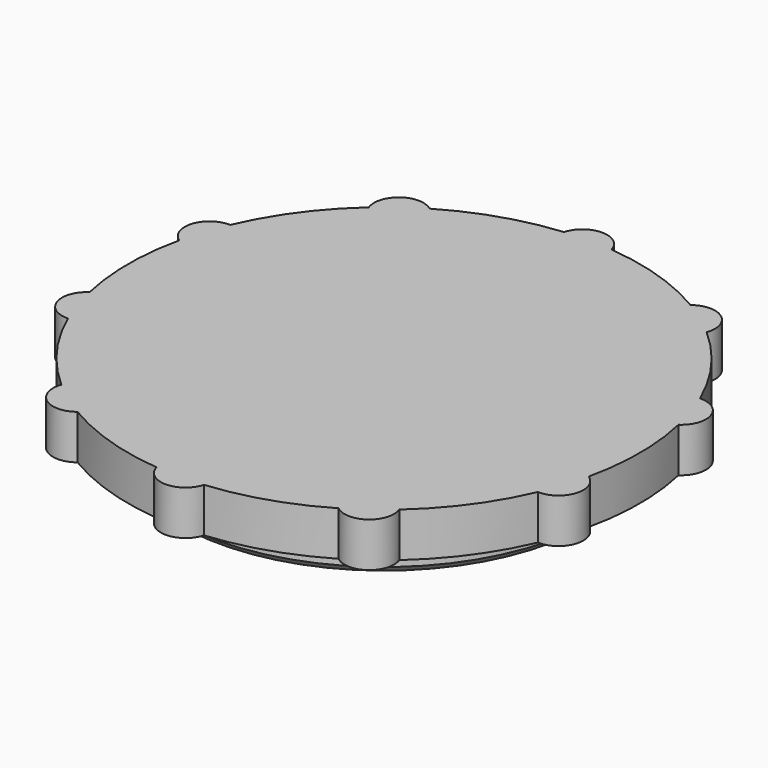
from build123d import *

# Parameters (mm, degrees)
F3_R            = 1.4097
F4_DEPTH        = 2.54
F4_COPIES_COUNT = 10
F5_SIZE         = 0.381


# Not quite as in the source:
# - a pattern or mirror of a feature is missing from the dataset's text; its kind, count and spacing are read off the source's solid


with BuildPart() as f2:
    # F1 (on Front) → F2 (revolve)
    with BuildSketch(Plane.XZ):
        Polygon((-14.605, 0), (-12.0904, 0), (-12.0904, -2.032), (-10.5791, -2.032), (-10.5791, 0), (-8.763, 0), (-7.874, 1.524), (0, 1.524), (0, 2.54), (-14.605, 2.54), align=None)
    revolve(axis=Axis((0, 0, -1.27), (0, 0, -1)))

    # F3 (on face) → F4 (join, through all)
    with BuildSketch(Plane.XY.offset(2.54)):
        with Locations((0, 14.1607994729)):
            Circle(F3_R)
    f4 = extrude(amount=-F4_DEPTH)

    # F4_copies: F4 ×10 about axis
    f4_copies_axis = Axis((0, 0, 0), (0, 0, 1))
    for i in range(1, F4_COPIES_COUNT):
        add(f4.rotate(f4_copies_axis, i * 360 / F4_COPIES_COUNT))

    # F5
    f5_edges = [f2.edges().sort_by_distance(p)[0] for p in [
        (12.0904, 0, -2.032),
    ]]
    chamfer(f5_edges, length=F5_SIZE)


solid = f2.part
